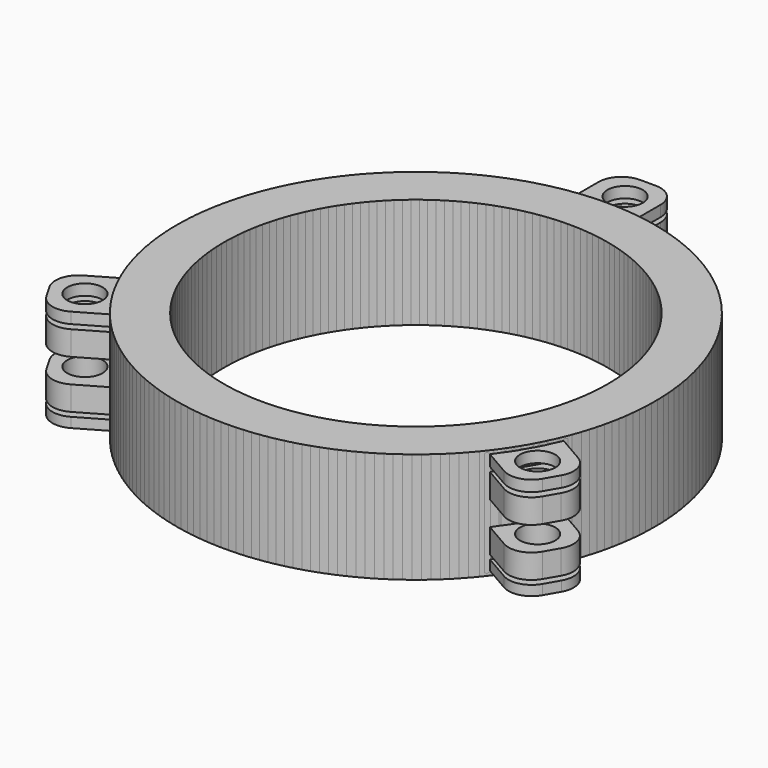
from build123d import *

# Parameters (mm, degrees)
F0_R     = 13.7469031818
F0_R_2   = 11.049
F1_DEPTH = 6.35
F3_START = -13.462
F2_W     = 3.5558892414
F2_H     = 1.397
F2_H_2   = 1.3914707582
F2_W_2   = 3.5618193036
F2_H_3   = 0.5705402
F2_H_4   = 0.6316690706
F3_DEPTH = 3.2512
F4_R     = 1.016
F5_DEPTH = 25.4
F6_R     = 1.3208
F7_COUNT = 3


# Not quite as in the source:
# - a feature names something its author has since deleted; it is built from what else it names


with BuildPart() as f1:
    # F0 (on Top) → F1 (new body)
    with BuildSketch(Plane.XY):
        Circle(F0_R)
        Circle(F0_R_2, mode=Mode.SUBTRACT)
    extrude(amount=F1_DEPTH)

    # F2 (on Front) → F3 (join)
    with BuildSketch(Plane.XZ.offset(F3_START)):
        with Locations((-0.0219139216, 4.5555063916)):
            Rectangle(F2_W, F2_H)
        with Locations((-0.0219139216, 1.7642710125)):
            Rectangle(F2_W, F2_H_2)
        with Locations((-0.0248789527, 0.5357988994)):
            Rectangle(F2_W_2, F2_H_3)
        with Locations((-0.0248789527, 5.8336711954)):
            Rectangle(F2_W_2, F2_H_4)
    extrude(amount=-F3_DEPTH)

    # F4 (on face) → F5 (cut)
    with BuildSketch(Plane(origin=(0, 0, 0.2505287994), x_dir=(1, 0, 0), z_dir=(0, 0, -1))):
        with Locations((0.0027344795, -15.0372548599)):
            Circle(F4_R)
    extrude(amount=-F5_DEPTH, mode=Mode.SUBTRACT)

    # F6
    f6_edges = [f1.edges().sort_by_distance(p)[0] for p in [
        (1.756031, 16.7132, 1.764271),
        (1.756031, 16.7132, 4.555506),
        (-1.799859, 16.7132, 4.555506),
        (-1.799859, 16.7132, 1.764271),
        (1.756031, 16.7132, 0.535799),
        (-1.805789, 16.7132, 0.535799),
        (-1.805789, 16.7132, 5.833671),
        (1.756031, 16.7132, 5.833671),
    ]]
    fillet(f6_edges, radius=F6_R)


with BuildPart() as f7_1:
    # F7: instance of F1
    add(f1.part.rotate(Axis((0, 0, 6.35), (0, 0, 1)), 1 * 360 / F7_COUNT))


with BuildPart() as f7_2:
    # F7: instance of F1
    add(f1.part.rotate(Axis((0, 0, 6.35), (0, 0, 1)), 2 * 360 / F7_COUNT))


solid = Compound([f1.part, f7_1.part, f7_2.part])
